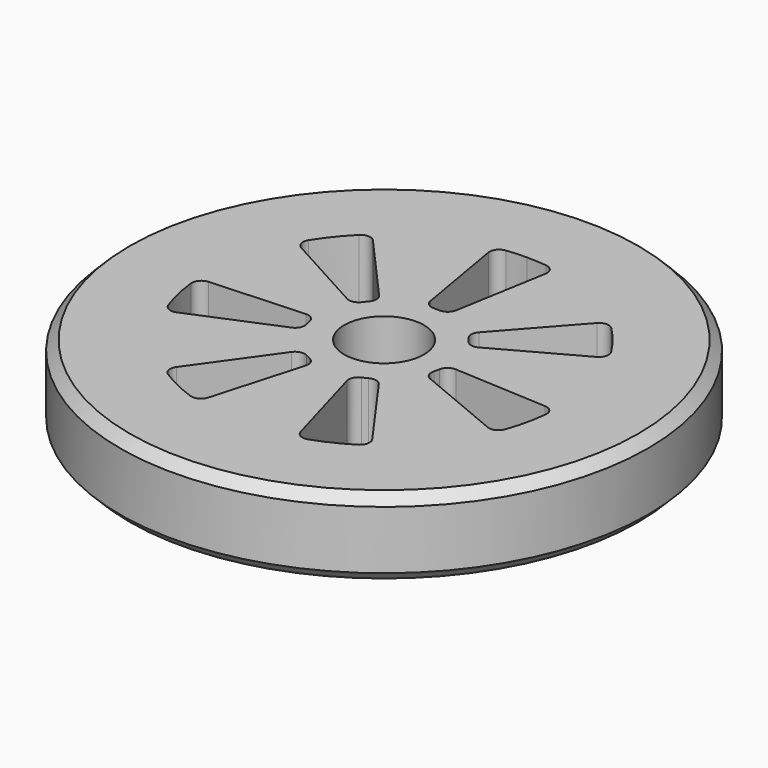
from build123d import *

# Parameters (mm, degrees)
F0_R      = 13.57391
F1_DEPTH  = 17
F3_DEPTH  = 1.5
F5_DEPTH  = 34
F6_R      = 15.57391
F6_R_2    = 13.57391
F7_DEPTH  = 1.5
F8_SIZE2  = 0.99999
F8_SIZE   = 1.99999
F9_R      = 1
F12_R     = 13.57391
F12_R_2   = 10.57391
F13_DEPTH = 2
F15_R     = 13.57391
F15_R_2   = 10.57391
F16_DEPTH = 2
F17_SIZE  = 0.49999
F18_R     = 19.7740128031
F18_R_2   = 13.57391
F19_DEPTH = 100
F20_DEPTH = 15
F10_R     = 13.57391
F10_R_2   = 10.32391
F21_DEPTH = 15
F22_R     = 2.05
F23_DEPTH = 25
F24_R     = 0.5


# Not quite as in the source:
# - a fillet or chamfer is up to 0.001 mm smaller than in the source, because OpenCascade refuses the exact size
# - a feature names something its author has since deleted; it is built from what else it names


with BuildPart() as f1:
    # F0 (on Top) → F1 (new body, symmetric)
    with BuildSketch(Plane.XY):
        Circle(F0_R)
    extrude(amount=F1_DEPTH, both=True)

    # F2 (on Top) → F3 (join, symmetric)
    with BuildSketch(Plane.XY):
        with BuildLine():
            Line((-8.8722387473, 10.27299432), (-13.094084175, 11.721231689))
            ThreePointArc((-13.094084175, 11.721231689), (-13.7398361081, 10.9571536638), (-14.3410637787, 10.1575687241))
            Line((-14.3410637787, 10.1575687241), (-11.9896877566, 6.3638369077))
            ThreePointArc((-11.9896877566, 6.3638369077), (-10.6125101782, 8.4631944563), (-8.8722387473, 10.27299432))
        make_face()
        with BuildLine():
            ThreePointArc((1, 17.5454356654), (0, 17.57391), (-1, 17.5454356654))
            Line((-1, 17.5454356654), (-2.5, 13.3417027657))
            ThreePointArc((-2.5, 13.3417027657), (0, 13.57391), (2.5, 13.3417027657))
            Line((2.5, 13.3417027657), (1, 17.5454356654))
        make_face()
        with BuildLine():
            Line((11.9896877566, 6.3638369077), (14.3410637787, 10.1575687241))
            ThreePointArc((14.3410637787, 10.1575687241), (13.7398361081, 10.9571536638), (13.094084175, 11.721231689))
            Line((13.094084175, 11.721231689), (8.8722387473, 10.27299432))
            ThreePointArc((8.8722387473, 10.27299432), (10.6125101782, 8.4631944563), (11.9896877566, 6.3638369077))
        make_face()
        with BuildLine():
            Line((12.4508960874, -5.4061279404), (16.8830140276, -4.8791546431))
            ThreePointArc((16.8830140276, -4.8791546431), (17.1332953852, -3.9105628665), (17.3280558955, -2.9292988187))
            Line((17.3280558955, -2.9292988187), (13.5635007572, -0.5314883795))
            ThreePointArc((13.5635007572, -0.5314883795), (13.2335837364, -3.0204791306), (12.4508960874, -5.4061279404))
        make_face()
        with BuildLine():
            Line((3.5363257124, -13.1051681845), (6.711710363, -16.2417750474))
            ThreePointArc((6.711710363, -16.2417750474), (7.6250337817, -15.8335457973), (8.5136480988, -15.3740075692))
            Line((8.5136480988, -15.3740075692), (8.0411700519, -10.9357494889))
            ThreePointArc((8.0411700519, -10.9357494889), (5.8894988252, -12.2296703257), (3.5363257124, -13.1051681845))
        make_face()
        with BuildLine():
            Line((-8.0411700519, -10.9357494889), (-8.5136480988, -15.3740075692))
            ThreePointArc((-8.5136480988, -15.3740075692), (-7.6250337817, -15.8335457973), (-6.711710363, -16.2417750474))
            Line((-6.711710363, -16.2417750474), (-3.5363257124, -13.1051681845))
            ThreePointArc((-3.5363257124, -13.1051681845), (-5.8894988252, -12.2296703257), (-8.0411700519, -10.9357494889))
        make_face()
        with BuildLine():
            Line((-13.5635007572, -0.5314883795), (-17.3280558955, -2.9292988187))
            ThreePointArc((-17.3280558955, -2.9292988187), (-17.1332953852, -3.9105628665), (-16.8830140276, -4.8791546431))
            Line((-16.8830140276, -4.8791546431), (-12.4508960874, -5.4061279404))
            ThreePointArc((-12.4508960874, -5.4061279404), (-13.2335837364, -3.0204791306), (-13.5635007572, -0.5314883795))
        make_face()
    extrude(amount=F3_DEPTH, both=True)

    # F4 (on face) → F5 (cut)
    with BuildSketch(Plane.XY.offset(17)):
        with BuildLine():
            ThreePointArc((-0.5774653997, 3.3439831422), (-0.2897912953, 3.3810812691), (0, 3.3934775))
            Line((0, 3.3934775), (0, 6.786955))
            Line((0, 6.786955), (0, 9.1804325))
            ThreePointArc((0, 9.1804325), (-0.7839773287, 9.1468967653), (-1.5622269849, 9.0465345705))
            Line((-1.5622269849, 9.0465345705), (-0.5774653997, 3.3439831422))
        make_face()
        with BuildLine():
            Line((0, 6.786955), (0, 3.3934775))
            ThreePointArc((0, 3.3934775), (0.2897912953, 3.3810812691), (0.5774653997, 3.3439831422))
            Line((0.5774653997, 3.3439831422), (1.5622269849, 9.0465345705))
            ThreePointArc((1.5622269849, 9.0465345705), (0.7839773287, 9.1468967653), (0, 9.1804325))
            Line((0, 9.1804325), (0, 6.786955))
        make_face()
        Polygon((-1.2990381057, 0.7133780277), (0, 0), (-0.8810810246, 0.9913076333), (-1.2990381057, 0.75), align=None)
        Polygon((-0.8810810246, 0.9913076333), (0, 0), (-0.2355474293, 1.3640066283), align=None)
        Polygon((-0.2355474293, 1.3640066283), (0, 0), (0, 1.5), align=None)
        Polygon((0, 1.5), (0, 0), (0.2355474293, 1.3640066283), align=None)
        Polygon((0.2355474293, 1.3640066283), (0, 0), (0.8810810246, 0.9913076333), align=None)
        Polygon((0.8810810246, 0.9913076333), (0, 0), (1.2990381057, 0.7133780277), (1.2990381057, 0.75), align=None)
        Polygon((1.2990381057, -0.5421957037), (0, 0), (0.7580809189, -1.0623217774), (1.2990381057, -0.75), align=None)
        Polygon((0.3672856493, -1.2879475315), (0, 0), (-0.3672856493, -1.2879475315), (0, -1.5), align=None)
        Polygon((-0.7580809189, -1.0623217774), (0, 0), (-1.2990381057, -0.5421957037), (-1.2990381057, -0.75), align=None)
        with BuildLine():
            Line((-8.0468981277, 4.4190238073), (-2.974475085, 1.6334587572))
            ThreePointArc((-2.974475085, 1.6334587572), (-2.6531275445, 2.1157986141), (-2.2543875098, 2.5364200163))
            Line((-2.2543875098, 2.5364200163), (-6.0988329412, 6.8618202864))
            ThreePointArc((-6.0988329412, 6.8618202864), (-7.1775511512, 5.7239060404), (-8.0468981277, 4.4190238073))
        make_face()
        with BuildLine():
            Line((6.0988329412, 6.8618202864), (2.2543875098, 2.5364200163))
            ThreePointArc((2.2543875098, 2.5364200163), (2.6531275445, 2.1157986141), (2.974475085, 1.6334587572))
            Line((2.974475085, 1.6334587572), (8.0468981277, 4.4190238073))
            ThreePointArc((8.0468981277, 4.4190238073), (7.1775511512, 5.7239060404), (6.0988329412, 6.8618202864))
        make_face()
        with BuildLine():
            Line((9.167347269, -0.489984629), (3.3886406432, -0.1811191154))
            ThreePointArc((3.3886406432, -0.1811191154), (3.3083959341, -0.7551197827), (3.1316443631, -1.3070933884))
            Line((3.1316443631, -1.3070933884), (8.4720908536, -3.5361020144))
            ThreePointArc((8.4720908536, -3.5361020144), (8.9502598902, -2.042838414), (9.167347269, -0.489984629))
        make_face()
        with BuildLine():
            Line((-8.4720908536, -3.5361020144), (-3.1316443631, -1.3070933884))
            ThreePointArc((-3.1316443631, -1.3070933884), (-3.3083959341, -0.7551197827), (-3.3886406432, -0.1811191154))
            Line((-3.3886406432, -0.1811191154), (-9.167347269, -0.489984629))
            ThreePointArc((-9.167347269, -0.489984629), (-8.9502598902, -2.042838414), (-8.4720908536, -3.5361020144))
        make_face()
        with BuildLine():
            Line((-2.5176263675, -8.8284708959), (-0.9306215619, -3.2633775527))
            ThreePointArc((-0.9306215619, -3.2633775527), (-1.4723747063, -3.0574175814), (-1.9711782567, -2.7622718591))
            Line((-1.9711782567, -2.7622718591), (-5.3326621235, -7.4728211249))
            ThreePointArc((-5.3326621235, -7.4728211249), (-3.9832403798, -8.2712838764), (-2.5176263675, -8.8284708959))
        make_face()
        with BuildLine():
            Line((5.3326621235, -7.4728211249), (1.9711782567, -2.7622718591))
            ThreePointArc((1.9711782567, -2.7622718591), (1.4723747063, -3.0574175814), (0.9306215619, -3.2633775527))
            Line((0.9306215619, -3.2633775527), (2.5176263675, -8.8284708959))
            ThreePointArc((2.5176263675, -8.8284708959), (3.9832403798, -8.2712838764), (5.3326621235, -7.4728211249))
        make_face()
    extrude(amount=-F5_DEPTH, mode=Mode.SUBTRACT)

    # F6 (on face) → F7 (join)
    with BuildSketch(Plane(origin=(0, 0, -17), x_dir=(1, 0, 0), z_dir=(0, 0, -1))):
        Circle(F6_R)
        Circle(F6_R_2, mode=Mode.SUBTRACT)
    extrude(amount=-F7_DEPTH)

    # F8 (size 2 and 1 in the source; OpenCascade refuses exactly that, so slightly less here)
    f8_edges = [f1.edges().sort_by_distance(p)[0] for p in [
        (-15.57391, 0, -15.5),
    ]]
    f8_side = f1.faces().sort_by_distance((-15.133413, 0, -15.5))[0]
    chamfer(f8_edges, length=F8_SIZE, length2=F8_SIZE2, reference=f8_side)

    # F9
    f9_edges = [f1.edges().sort_by_distance(p)[0] for p in [
        (14.341064, 10.157569, 0),
        (13.094084, 11.721232, 0),
        (1, 17.545436, 0),
        (-1, 17.545436, 0),
        (-13.094084, 11.721232, 0),
        (-14.341064, 10.157569, 0),
        (-17.328056, -2.929299, 0),
        (-16.883014, -4.879155, 0),
        (-8.513648, -15.374008, 0),
        (-6.71171, -16.241775, 0),
        (6.71171, -16.241775, 0),
        (8.513648, -15.374008, 0),
        (16.883014, -4.879155, 0),
        (17.328056, -2.929299, 0),
    ]]
    fillet(f9_edges, radius=F9_R)

    # F12 (on offset) → F13 (cut)
    with BuildSketch(Plane.XY.offset(2)):
        Circle(F12_R)
        Circle(F12_R_2, mode=Mode.SUBTRACT)
    extrude(amount=F13_DEPTH, mode=Mode.SUBTRACT)

    # F15 (on offset) → F16 (cut)
    with BuildSketch(Plane(origin=(0, 0, -2), x_dir=(1, 0, 0), z_dir=(0, 0, -1))):
        Circle(F15_R)
        Circle(F15_R_2, mode=Mode.SUBTRACT)
    extrude(amount=F16_DEPTH, mode=Mode.SUBTRACT)

    # F17 (size 0.5 in the source; OpenCascade refuses exactly that, so slightly less here)
    f17_edges = [f1.edges().sort_by_distance(p)[0] for p in [
        (-13.57391, 0, -4),
        (-13.57391, 0, -2),
        (-13.57391, 0, 2),
        (-13.57391, 0, 4),
    ]]
    chamfer(f17_edges, length=F17_SIZE)

    # F18 (on face) → F19 (cut)
    with BuildSketch(Plane.XY.offset(17)):
        Circle(F18_R)
        Circle(F18_R_2, mode=Mode.SUBTRACT)
    extrude(amount=-F19_DEPTH, mode=Mode.SUBTRACT)

    # F20 (cut): a face of the model
    f20_faces = [f1.faces().sort_by_distance(p)[0] for p in [
        (-13.1899818477, 0, 17),
    ]]
    extrude(f20_faces, amount=-F20_DEPTH, mode=Mode.SUBTRACT)

    # F10 (on face) → F21 (cut)
    with BuildSketch(Plane(origin=(0, 0, -17), x_dir=(1, 0, 0), z_dir=(0, 0, -1))):
        Circle(F10_R)
        Circle(F10_R_2, mode=Mode.SUBTRACT)
        Circle(F10_R_2)
        with BuildLine():
            Line((-2.2543875098, -2.5364200163), (-6.0988329412, -6.8618202864))
            ThreePointArc((-6.0988329412, -6.8618202864), (-7.1775511512, -5.7239060404), (-8.0468981277, -4.4190238073))
            Line((-8.0468981277, -4.4190238073), (-2.974475085, -1.6334587572))
            ThreePointArc((-2.974475085, -1.6334587572), (-2.6531275445, -2.1157986141), (-2.2543875098, -2.5364200163))
        make_face(mode=Mode.SUBTRACT)
        with BuildLine():
            ThreePointArc((-0.5774653997, -3.3439831422), (0, -3.3934775), (0.5774653997, -3.3439831422))
            Line((0.5774653997, -3.3439831422), (1.5622269849, -9.0465345705))
            ThreePointArc((1.5622269849, -9.0465345705), (0, -9.1804325), (-1.5622269849, -9.0465345705))
            Line((-1.5622269849, -9.0465345705), (-0.5774653997, -3.3439831422))
        make_face(mode=Mode.SUBTRACT)
        with BuildLine():
            ThreePointArc((8.0468981277, -4.4190238073), (7.1775511512, -5.7239060404), (6.0988329412, -6.8618202864))
            Line((6.0988329412, -6.8618202864), (2.2543875098, -2.5364200163))
            ThreePointArc((2.2543875098, -2.5364200163), (2.6531275445, -2.1157986141), (2.974475085, -1.6334587572))
            Line((2.974475085, -1.6334587572), (8.0468981277, -4.4190238073))
        make_face(mode=Mode.SUBTRACT)
        Polygon((-1.2990381057, -0.7133780277), (0, 0), (1.2990381057, -0.7133780277), (1.2990381057, -0.75), (0, -1.5), (-1.2990381057, -0.75), align=None, mode=Mode.SUBTRACT)
        with BuildLine():
            Line((-3.3886406432, 0.1811191154), (-9.167347269, 0.489984629))
            ThreePointArc((-9.167347269, 0.489984629), (-8.9502598902, 2.042838414), (-8.4720908536, 3.5361020144))
            Line((-8.4720908536, 3.5361020144), (-3.1316443631, 1.3070933884))
            ThreePointArc((-3.1316443631, 1.3070933884), (-3.3083959341, 0.7551197827), (-3.3886406432, 0.1811191154))
        make_face(mode=Mode.SUBTRACT)
        Polygon((-0.7580809189, 1.0623217774), (0, 0), (-1.2990381057, 0.5421957037), (-1.2990381057, 0.75), align=None, mode=Mode.SUBTRACT)
        with BuildLine():
            Line((-1.9711782567, 2.7622718591), (-5.3326621235, 7.4728211249))
            ThreePointArc((-5.3326621235, 7.4728211249), (-3.9832403798, 8.2712838764), (-2.5176263675, 8.8284708959))
            Line((-2.5176263675, 8.8284708959), (-0.9306215619, 3.2633775527))
            ThreePointArc((-0.9306215619, 3.2633775527), (-1.4723747063, 3.0574175814), (-1.9711782567, 2.7622718591))
        make_face(mode=Mode.SUBTRACT)
        Polygon((0.3672856493, 1.2879475315), (0, 0), (-0.3672856493, 1.2879475315), (0, 1.5), align=None, mode=Mode.SUBTRACT)
        Polygon((1.2990381057, 0.5421957037), (0, 0), (0.7580809189, 1.0623217774), (1.2990381057, 0.75), align=None, mode=Mode.SUBTRACT)
        with BuildLine():
            Line((3.1316443631, 1.3070933884), (8.4720908536, 3.5361020144))
            ThreePointArc((8.4720908536, 3.5361020144), (8.9502598902, 2.042838414), (9.167347269, 0.489984629))
            Line((9.167347269, 0.489984629), (3.3886406432, 0.1811191154))
            ThreePointArc((3.3886406432, 0.1811191154), (3.3083959341, 0.7551197827), (3.1316443631, 1.3070933884))
        make_face(mode=Mode.SUBTRACT)
        with BuildLine():
            Line((0.9306215619, 3.2633775527), (2.5176263675, 8.8284708959))
            ThreePointArc((2.5176263675, 8.8284708959), (3.9832403798, 8.2712838764), (5.3326621235, 7.4728211249))
            Line((5.3326621235, 7.4728211249), (1.9711782567, 2.7622718591))
            ThreePointArc((1.9711782567, 2.7622718591), (1.4723747063, 3.0574175814), (0.9306215619, 3.2633775527))
        make_face(mode=Mode.SUBTRACT)
    extrude(amount=-F21_DEPTH, mode=Mode.SUBTRACT)

    # F22 (on face) → F23 (cut)
    with BuildSketch(Plane(origin=(0, 0, -2), x_dir=(1, 0, 0), z_dir=(0, 0, -1))):
        Circle(F22_R)
        Polygon((-1.2990381057, -0.7133780277), (0, 0), (1.2990381057, -0.7133780277), (1.2990381057, -0.75), (0, -1.5), (-1.2990381057, -0.75), align=None, mode=Mode.SUBTRACT)
        Polygon((-0.7580809189, 1.0623217774), (0, 0), (-1.2990381057, 0.5421957037), (-1.2990381057, 0.75), align=None, mode=Mode.SUBTRACT)
        Polygon((0.3672856493, 1.2879475315), (0, 0), (-0.3672856493, 1.2879475315), (0, 1.5), align=None, mode=Mode.SUBTRACT)
        Polygon((1.2990381057, 0.5421957037), (0, 0), (0.7580809189, 1.0623217774), (1.2990381057, 0.75), align=None, mode=Mode.SUBTRACT)
    extrude(amount=-F23_DEPTH, mode=Mode.SUBTRACT)

    # F24
    f24_edges = [f1.edges().sort_by_distance(p)[0] for p in [
        (-1.971178, -2.762272, 0),
        (-0.930622, -3.263378, 0),
        (1.971178, -2.762272, 0),
        (0.930622, -3.263378, 0),
        (3.388641, -0.181119, 0),
        (3.131644, -1.307093, 0),
        (2.254388, 2.53642, 0),
        (2.974475, 1.633459, 0),
        (-0.577465, 3.343983, 0),
        (0.577465, 3.343983, 0),
        (-2.254388, 2.53642, 0),
        (-2.974475, 1.633459, 0),
        (-3.388641, -0.181119, 0),
        (-3.131644, -1.307093, 0),
        (-9.167347, -0.489985, 0),
        (-8.472091, -3.536102, 0),
        (-8.046898, 4.419024, 0),
        (-6.098833, 6.86182, 0),
        (-1.562227, 9.046535, 0),
        (1.562227, 9.046535, 0),
        (6.098833, 6.86182, 0),
        (8.046898, 4.419024, 0),
        (9.167347, -0.489985, 0),
        (8.472091, -3.536102, 0),
        (5.332662, -7.472821, 0),
        (2.517626, -8.828471, 0),
        (-2.517626, -8.828471, 0),
        (-5.332662, -7.472821, 0),
    ]]
    fillet(f24_edges, radius=F24_R)


solid = f1.part
